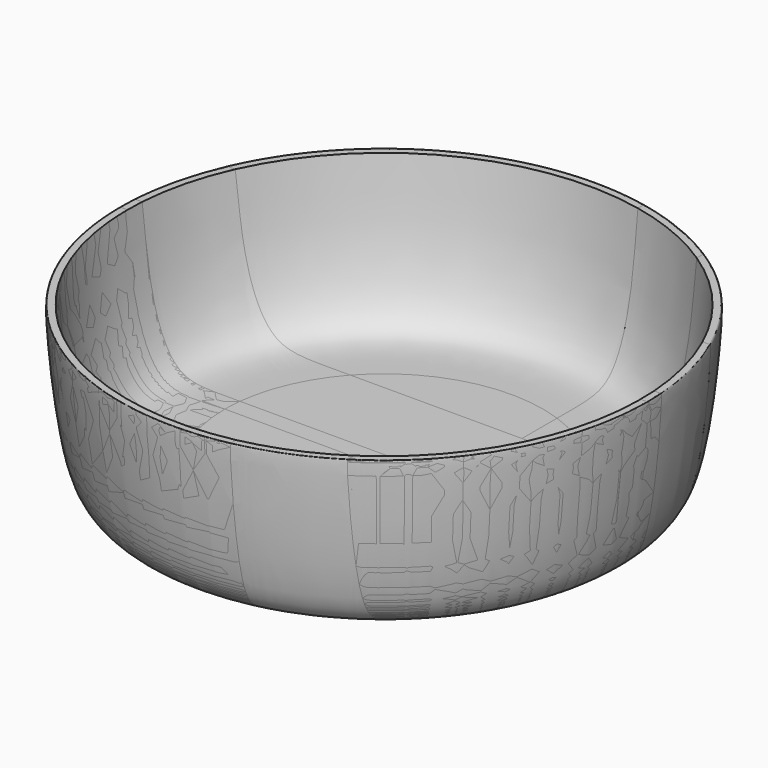
from build123d import *

# Parameters (mm, degrees)
F0_W      = 90
F0_H      = 45
F1_DEPTH  = 50
F0_W_2    = 25
F2_DEPTH  = 50
F0_W_3    = 45
F3_DEPTH  = 50
F4_DEPTH  = 50
F0_H_2    = 5
F0_H_3    = 75
F5_DEPTH  = 50
F6_DEPTH  = 50
F7_DEPTH  = 50
F8_DEPTH  = 50
F9_DEPTH  = 50
F10_DEPTH = 50
F11_DEPTH = 50
F12_DEPTH = 50
F13_W     = 15
F13_H     = 4.0908760428


# Not quite as in the source:
# - a feature names something its author has since deleted; it is built from what else it names


with BuildPart() as f1:
    # F0 (on Top) → F1 (new body)
    with BuildSketch(Plane.XY):
        with Locations((45, 47.5)):
            Rectangle(F0_W, F0_H)
    extrude(amount=F1_DEPTH)


with BuildPart() as f2:
    # F0 (on Top) → F2 (new body)
    with BuildSketch(Plane.XY):
        with Locations((102.5, 47.5)):
            Rectangle(F0_W_2, F0_H)
    extrude(amount=F2_DEPTH)


with BuildPart() as f3:
    # F0 (on Top) → F3 (new body)
    with BuildSketch(Plane.XY):
        with Locations((137.5, 47.5)):
            Rectangle(F0_W_3, F0_H)
    extrude(amount=F3_DEPTH)


with BuildPart() as f4:
    # F0 (on Top) → F4 (new body)
    with BuildSketch(Plane.XY):
        Polygon((0, 25), (0, 0), (90, 0), (100, 0), (115, 0), (125, 0), (160, 0), (160, 25), (115, 25), (90, 25), align=None)
    extrude(amount=F4_DEPTH)


with BuildPart() as f5:
    # F0 (on Top) → F5 (new body)
    with BuildSketch(Plane.XY):
        with Locations((45, -2.5)):
            Rectangle(F0_W, F0_H_2)
        with Locations((45, -42.5)):
            Rectangle(F0_W, F0_H_3)
    extrude(amount=F5_DEPTH)


with BuildPart() as f5b:
    # F0 (on Top) → F5, piece 2 (new body)
    with BuildSketch(Plane.XY):
        Polygon((115, 0), (115, -5), (160, -5), (160, 0), (125, 0), align=None)
        with Locations((137.5, -42.5)):
            Rectangle(F0_W_3, F0_H_3)
    extrude(amount=F5_DEPTH)


with BuildPart() as f6:
    # F0 (on Top) → F6 (new body)
    with BuildSketch(Plane.XY):
        Polygon((100, 0), (90, 0), (90, -5), (115, -5), (115, 0), align=None)
        with Locations((102.5, -42.5)):
            Rectangle(F0_W_2, F0_H_3)
    extrude(amount=F6_DEPTH)


with BuildPart() as f7:
    # F0 (on Top) → F7 (new body)
    with BuildSketch(Plane.XY):
        with Locations((45, -2.5)):
            Rectangle(F0_W, F0_H_2)
    extrude(amount=F7_DEPTH)


with BuildPart() as f8:
    # F0 (on Top) → F8 (new body)
    with BuildSketch(Plane.XY):
        Polygon((100, 0), (90, 0), (90, -5), (115, -5), (115, 0), align=None)
    extrude(amount=F8_DEPTH)


with BuildPart() as f9:
    # F0 (on Top) → F9 (new body)
    with BuildSketch(Plane.XY):
        Polygon((115, 0), (115, -5), (160, -5), (160, 0), (125, 0), align=None)
    extrude(amount=F9_DEPTH)


with BuildPart() as f10:
    # F0 (on Top) → F10 (new body)
    with BuildSketch(Plane.XY):
        with Locations((45, -42.5)):
            Rectangle(F0_W, F0_H_3)
    extrude(amount=F10_DEPTH)


with BuildPart() as f11:
    # F0 (on Top) → F11 (new body)
    with BuildSketch(Plane.XY):
        with Locations((102.5, -42.5)):
            Rectangle(F0_W_2, F0_H_3)
    extrude(amount=F11_DEPTH)


with BuildPart() as f12:
    # F0 (on Top) → F12 (new body)
    with BuildSketch(Plane.XY):
        with Locations((137.5, -42.5)):
            Rectangle(F0_W_3, F0_H_3)
    extrude(amount=F12_DEPTH)


with BuildPart() as f14_tool:
    # F13 (on face) → F14 (revolve)
    with BuildSketch(Plane.XZ.offset(5)):
        with Locations((82.5, 6.0454380214)):
            Rectangle(F13_W, F13_H)
        with BuildLine():
            Line((90, 8.0908760428), (90, 4))
            Line((90, 4), (101, 4))
            Line((101, 4), (99.2046818137, 0))
            Line((99.2046818137, 0), (119.2046818137, 0))
            add(Edge.make_bspline(
                [(119.2046818137, 0), (126.2493979814, 0.7732794744), (138.9863898746, 2.1713846872), (147.3157369656, 10.0187020689), (150.1161102275, 49.1551977245), (149.4910913046, 48.7744319361), (149.4630426168, 48.7573444843)],
                knots=[0, 0, 0, 0, 0.3078185803, 0.5565423317, 0.9800991534, 1, 1, 1, 1], degree=3))
            Line((149.4630426168, 48.7573444843), (147.5605070591, 48.7573444843))
            add(Edge.make_bspline(
                [(120, 8.0908760428), (129.3039530386, 8.0908760428), (138.5548123003, 7.3831138404), (145.7109533824, 27.1683688424), (146.7088145562, 41.5130421868), (147.5605070591, 48.7573444843)],
                knots=[0, 0, 0, 0, 0.3205308098, 0.6379484552, 1, 1, 1, 1], degree=3))
            Line((120, 8.0908760428), (90, 8.0908760428))
        make_face()
    revolve(axis=Axis((75, -5, 22.4669491872), (0, 0, -1)))


with BuildPart() as f1_1:
    add(f1.part)

    # F14: intersect by f14_tool
    add(f14_tool.part, mode=Mode.INTERSECT)


with BuildPart() as f2_1:
    add(f2.part)

    # F14: intersect by f14_tool
    add(f14_tool.part, mode=Mode.INTERSECT)


with BuildPart() as f3_1:
    add(f3.part)

    # F14: intersect by f14_tool
    add(f14_tool.part, mode=Mode.INTERSECT)


with BuildPart() as f4_1:
    add(f4.part)

    # F14: intersect by f14_tool
    add(f14_tool.part, mode=Mode.INTERSECT)


with BuildPart() as f5_1:
    add(f5.part)

    # F14: intersect by f14_tool
    add(f14_tool.part, mode=Mode.INTERSECT)


with BuildPart() as f5b_1:
    add(f5b.part)

    # F14: intersect by f14_tool
    add(f14_tool.part, mode=Mode.INTERSECT)


with BuildPart() as f6_1:
    add(f6.part)

    # F14: intersect by f14_tool
    add(f14_tool.part, mode=Mode.INTERSECT)


with BuildPart() as f7_1:
    add(f7.part)

    # F14: intersect by f14_tool
    add(f14_tool.part, mode=Mode.INTERSECT)


with BuildPart() as f8_1:
    add(f8.part)

    # F14: intersect by f14_tool
    add(f14_tool.part, mode=Mode.INTERSECT)


with BuildPart() as f9_1:
    add(f9.part)

    # F14: intersect by f14_tool
    add(f14_tool.part, mode=Mode.INTERSECT)


with BuildPart() as f10_1:
    add(f10.part)

    # F14: intersect by f14_tool
    add(f14_tool.part, mode=Mode.INTERSECT)


with BuildPart() as f11_1:
    add(f11.part)

    # F14: intersect by f14_tool
    add(f14_tool.part, mode=Mode.INTERSECT)


with BuildPart() as f12_1:
    add(f12.part)

    # F14: intersect by f14_tool
    add(f14_tool.part, mode=Mode.INTERSECT)


solid = Compound([f1_1.part, f2_1.part, f3_1.part, f4_1.part, f5_1.part, f5b_1.part, f6_1.part, f7_1.part, f8_1.part, f9_1.part, f10_1.part, f11_1.part, f12_1.part])
